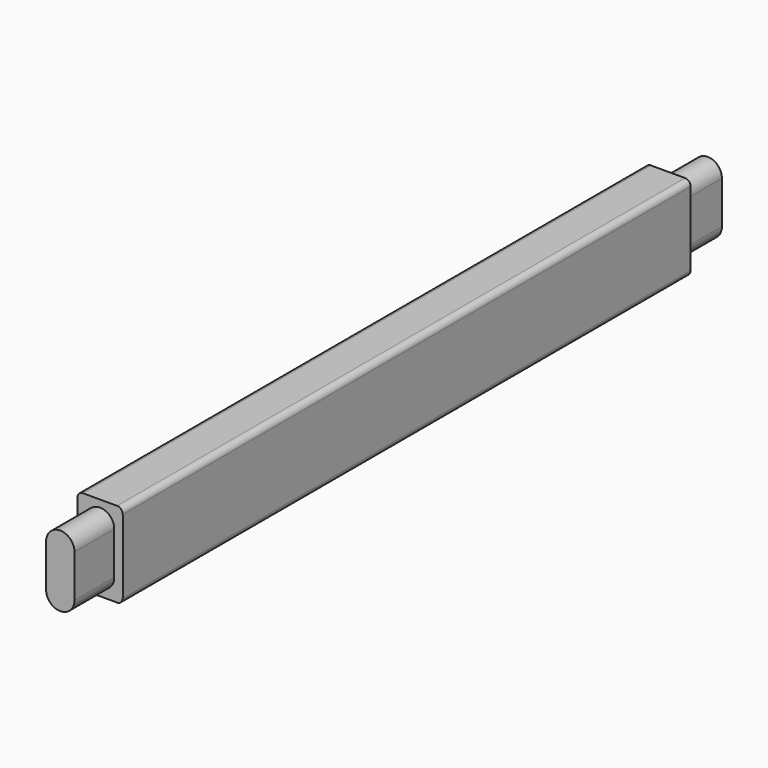
from build123d import *

# Parameters (mm, degrees)
F0_W          = 16
F0_H          = 30
F1_DEPTH      = 142.5
F1_DEPTH_BACK = 142.5
F2_W          = 16
F2_H          = 30
F3_DEPTH      = 17.5
F4_R          = 2


# Not quite as in the source:
# - a pattern or mirror of a feature is missing from the dataset's text; its kind, count and spacing are read off the source's solid


with BuildPart() as f1:
    # F0 (on Front) → F1 (new body, two sides)
    with BuildSketch(Plane.XZ) as f1_sk:
        Rectangle(F0_W, F0_H)
    extrude(amount=F1_DEPTH)
    extrude(f1_sk.sketch, amount=-F1_DEPTH_BACK)

    # F2 (on face) → F3 (cut)
    with BuildSketch(Plane.XZ.offset(142.5)):
        Rectangle(F2_W, F2_H)
        with BuildLine():
            ThreePointArc((5, -7.5), (0, -12.5), (-5, -7.5))
            Line((-5, -7.5), (-5, 7.5))
            ThreePointArc((-5, 7.5), (0, 12.5), (5, 7.5))
            Line((5, 7.5), (5, -7.5))
        make_face(mode=Mode.SUBTRACT)
    f3 = extrude(amount=-F3_DEPTH, mode=Mode.SUBTRACT)

    # F3_copies: F3 across plane
    add(f3.mirror(Plane.ZX), mode=Mode.SUBTRACT)

    # F4
    f4_edges = [f1.edges().sort_by_distance(p)[0] for p in [
        (-8, 0, 15),
        (8, 0, 15),
        (8, 0, -15),
        (-8, 0, -15),
    ]]
    fillet(f4_edges, radius=F4_R)


solid = f1.part
